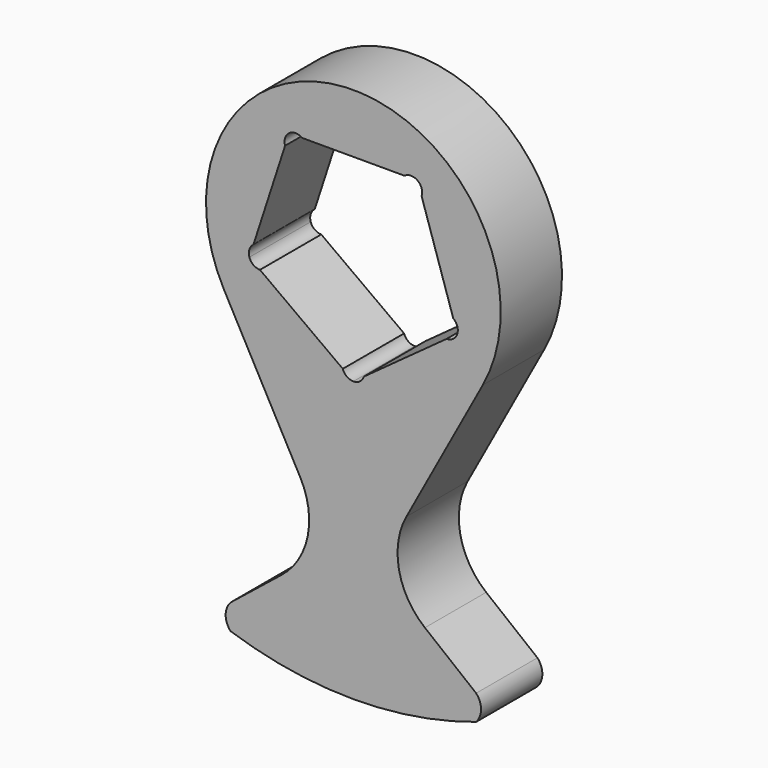
from build123d import *

# Parameters (mm, degrees)
F1_DEPTH = 39


with BuildPart() as f1:
    # F0 (on Front) → F1 (new body)
    with BuildSketch(Plane.XZ):
        with BuildLine():
            ThreePointArc((65.9112834496, -35.7869070195), (0, 75), (-65.9112834496, -35.7869070195))
            Line((-65.9112834496, -35.7869070195), (-26.9968870374, -107.4583093791))
            ThreePointArc((-26.9968870374, -107.4583093791), (-23.2346773471, -132.5123240584), (-36.426916686, -154.1415333488))
            Line((-36.426916686, -154.1415333488), (-62.5, -175))
            ThreePointArc((-62.5, -175), (-65, -181.4384772072), (-62.5, -187.8769544143))
            ThreePointArc((-62.5, -187.8769544143), (0, -198), (62.5, -187.8769544143))
            ThreePointArc((62.5, -187.8769544143), (65, -181.4384772072), (62.5, -175))
            Line((62.5, -175), (36.426916686, -154.1415333488))
            ThreePointArc((36.426916686, -154.1415333488), (23.2346773471, -132.5123240584), (26.9968870374, -107.4583093791))
            Line((26.9968870374, -107.4583093791), (65.9112834496, -35.7869070195))
        make_face()
        with BuildLine():
            ThreePointArc((-34.7452932117, 38.6880420754), (-34.7452932117, 42.1772066019), (-32.6944137602, 45))
            ThreePointArc((-32.6944137602, 45), (-29.3760211009, 46.0782111348), (-26.0576284416, 45))
            ThreePointArc((-26.0576284416, 45), (0, 52), (26.0576284416, 45))
            ThreePointArc((26.0576284416, 45), (29.3760211009, 46.0782111348), (32.6944137602, 45))
            ThreePointArc((32.6944137602, 45), (34.7452932117, 42.1772066019), (34.7452932117, 38.6880420754))
            ThreePointArc((34.7452932117, 38.6880420754), (47.4908162017, 21.1807076486), (52, 0))
            ThreePointArc((52, 0), (51.7116488291, -5.4685807459), (50.8497932548, -10.8765125817))
            ThreePointArc((50.8497932548, -10.8765125817), (52.9006727063, -13.6993059798), (52.9006727063, -17.1884705063))
            ThreePointArc((52.9006727063, -17.1884705063), (50.8497932548, -20.0112639043), (47.5314005955, -21.0894750392))
            ThreePointArc((47.5314005955, -21.0894750392), (30.5648331192, -42.0688837075), (5.3692721108, -51.7220544546))
            ThreePointArc((5.3692721108, -51.7220544546), (3.3183926593, -54.5448478526), (0, -55.6230589875))
            ThreePointArc((0, -55.6230589875), (-3.3183926593, -54.5448478526), (-5.3692721108, -51.7220544546))
            ThreePointArc((-5.3692721108, -51.7220544546), (-30.5648331192, -42.0688837075), (-47.5314005955, -21.0894750392))
            ThreePointArc((-47.5314005955, -21.0894750392), (-50.8497932548, -20.0112639043), (-52.9006727063, -17.1884705063))
            ThreePointArc((-52.9006727063, -17.1884705063), (-52.9006727063, -13.6993059798), (-50.8497932548, -10.8765125817))
            ThreePointArc((-50.8497932548, -10.8765125817), (-49.4549388473, 16.0688837075), (-34.7452932117, 38.6880420754))
        make_face(mode=Mode.SUBTRACT)
        with BuildLine():
            ThreePointArc((26.0576284416, 45), (0, 52), (-26.0576284416, 45))
            Line((-26.0576284416, 45), (26.0576284416, 45))
        make_face()
        with BuildLine():
            Line((-50.8497932548, -10.8765125817), (-34.7452932117, 38.6880420754))
            ThreePointArc((-34.7452932117, 38.6880420754), (-49.4549388473, 16.0688837075), (-50.8497932548, -10.8765125817))
        make_face()
        with BuildLine():
            ThreePointArc((52, 0), (47.4908162017, 21.1807076486), (34.7452932117, 38.6880420754))
            Line((34.7452932117, 38.6880420754), (50.8497932548, -10.8765125817))
            ThreePointArc((50.8497932548, -10.8765125817), (51.7116488291, -5.4685807459), (52, 0))
        make_face()
        with BuildLine():
            Line((-5.3692721108, -51.7220544546), (-47.5314005955, -21.0894750392))
            ThreePointArc((-47.5314005955, -21.0894750392), (-30.5648331192, -42.0688837075), (-5.3692721108, -51.7220544546))
        make_face()
        with BuildLine():
            ThreePointArc((5.3692721108, -51.7220544546), (30.5648331192, -42.0688837075), (47.5314005955, -21.0894750392))
            Line((47.5314005955, -21.0894750392), (5.3692721108, -51.7220544546))
        make_face()
    extrude(amount=F1_DEPTH)


solid = f1.part
